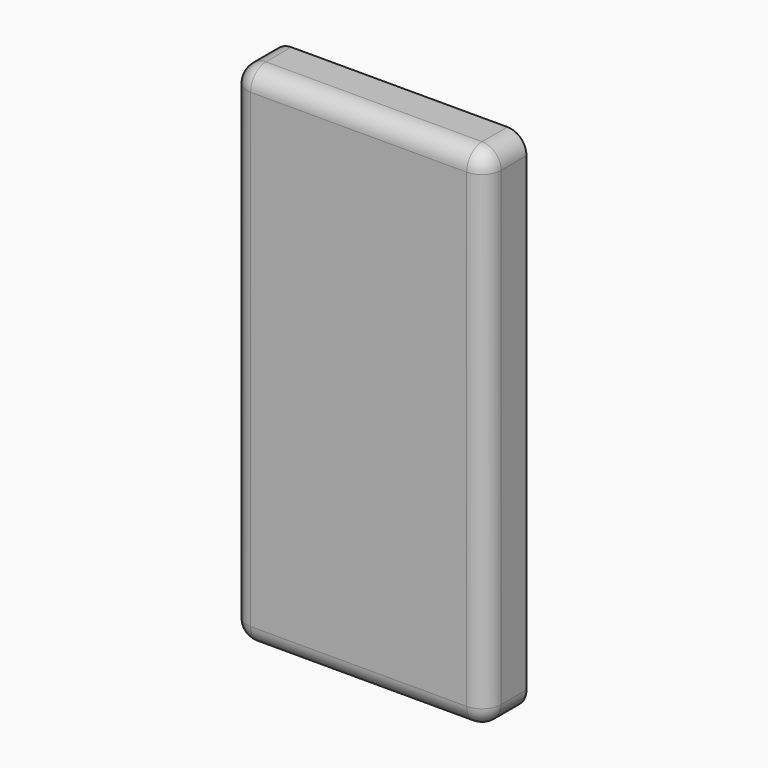
from build123d import *

# Parameters (mm, degrees)
F0_W     = 20
F0_H     = 40
F0_R     = 2.5
F3_DEPTH = 4
F4_R     = 1.5


# Not quite as in the source:
# - the program builds the solid bodies; features that only make, move or delete a surface that nothing else refers to are left out


with BuildPart() as f3:
    # F0 (on Front) → F3 (new body)
    with BuildSketch(Plane.XZ):
        with Locations((10, -20)):
            Rectangle(F0_W, F0_H)
        with Locations((10, -29.9999993294)):
            Circle(F0_R, mode=Mode.SUBTRACT)
        with Locations((10, -10)):
            Circle(F0_R, mode=Mode.SUBTRACT)
        with Locations((10, -10)):
            Circle(F0_R)
        with Locations((10, -29.9999993294)):
            Circle(F0_R)
    extrude(amount=F3_DEPTH)

    # F4
    f4_edges = [f3.edges().sort_by_distance(p)[0] for p in [
        (0, -2, 0),
        (0, -4, -20),
        (0, -2, -40),
        (10, -4, -40),
        (20, -2, -40),
        (20, -4, -20),
        (10, -4, 0),
        (20, -2, 0),
    ]]
    fillet(f4_edges, radius=F4_R)


solid = f3.part
